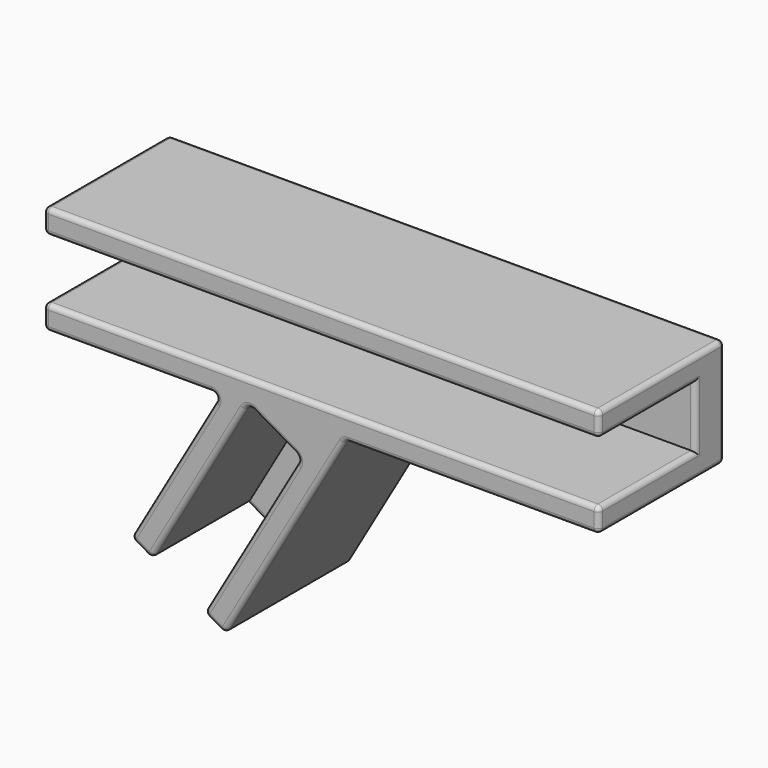
from build123d import *

# Parameters (mm, degrees)
F1_DEPTH      = 12.7
F0_W          = 58.42
F0_H          = 2.54
F0_H_2        = 6.35
F2_DEPTH      = 3.81
F4_T1_DEPTH   = 16.51
F4_T3_DEPTH   = 57.404
F4_T5_DEPTH   = 12.192
F4_T7_DEPTH   = 13.97
F4_T9_DEPTH   = 19.05
F4_T11_DEPTH  = 12.192
F4_T13_DEPTH  = 1.524
F4_T15_DEPTH  = 15.494
F4_T17_DEPTH  = 3.302
F4_T19_DEPTH  = 6.35
F4_T21_DEPTH  = 3.302
F4_T23_DEPTH  = 19.177
F4_T25_DEPTH  = 5.08
F4_T27_DEPTH  = 19.177
F4_T29_DEPTH  = 3.302
F4_T31_DEPTH  = 6.35
F4_S35_W      = 0.508
F4_S35_H      = 0.508
F4_T36_DEPTH  = 0.508
F4_S41_W      = 0.508
F4_S41_H      = 0.508
F4_T42_DEPTH  = 0.508
F4_S47_W      = 0.508
F4_S47_H      = 0.508
F4_T48_DEPTH  = 0.508
F4_S53_W      = 0.508
F4_S53_H      = 0.508
F4_T54_DEPTH  = 0.508
F4_S59_W      = 0.508
F4_S59_H      = 0.508
F4_T60_DEPTH  = 0.508
F4_S65_W      = 0.508
F4_S65_H      = 0.508
F4_T66_DEPTH  = 0.508
F4_S71_W      = 0.508
F4_S71_H      = 0.508
F4_T72_DEPTH  = 0.508
F4_S77_W      = 0.508
F4_S77_H      = 0.508
F4_T78_DEPTH  = 0.508
F4_S83_W      = 0.508
F4_S83_H      = 0.508
F4_T84_DEPTH  = 0.508
F4_S89_W      = 0.508
F4_S89_H      = 0.508
F4_T90_DEPTH  = 0.508
F4_T94_ANGLE  = 90
F4_T96_ANGLE  = 90
F4_T101_DEPTH = 13.462
F4_T105_DEPTH = 7.62
F4_T112_DEPTH = 13.462
F4_T116_DEPTH = 7.62
F4_T123_DEPTH = 13.462
F4_T127_DEPTH = 7.62
F4_T134_DEPTH = 7.62
F4_T138_DEPTH = 13.462
F4_T145_DEPTH = 13.462
F4_T149_DEPTH = 7.62
F4_T156_DEPTH = 7.62
F4_T160_DEPTH = 13.462
F4_T163_DEPTH = 17.1394104101
F4_T165_DEPTH = 17.4130046129
F4_T167_DEPTH = 24.5987060633
F4_T169_DEPTH = 25.8931866893
F4_T174_DEPTH = 0.508
F4_S179_W     = 0.508
F4_S179_H     = 0.508
F4_T180_DEPTH = 0.508
F4_S185_W     = 0.508
F4_S185_H     = 0.508
F4_T186_DEPTH = 0.508
F4_T192_DEPTH = 0.508
F4_S197_W     = 0.508
F4_S197_H     = 0.508
F4_T198_DEPTH = 0.508
F4_T204_DEPTH = 0.508
F4_T210_DEPTH = 0.508
F4_S215_W     = 0.508
F4_S215_H     = 0.508
F4_T216_DEPTH = 0.508
F4_T220_ANGLE = 120
F4_T222_ANGLE = 60
F4_T224_ANGLE = 60
F4_T226_ANGLE = 120


# Not quite as in the source:
# - a fillet or chamfer that OpenCascade refuses, or shapes differently, is made with other operations: its cross-section is extruded or revolved along the edge and cut away or added


with BuildPart() as f1:
    # F0 (on Front) → F1 (new body)
    with BuildSketch(Plane.XZ):
        with BuildLine():
            Line((29.21, -5.715), (29.21, -3.175))
            Line((29.21, -3.175), (-29.21, -3.175))
            Line((-29.21, -3.175), (-29.21, -5.715))
            Line((-29.21, -5.715), (-10.6827077797, -5.715))
            Line((-10.6827077797, -5.715), (-20.0831509913, -21.9970452561))
            Line((-20.0831509913, -21.9970452561), (-17.8834464656, -23.2670452561))
            Line((-17.8834464656, -23.2670452561), (-8.0409464656, -6.2193351826))
            ThreePointArc((-8.0409464656, -6.2193351826), (-7.6553704279, -5.9234722829), (-7.1735203342, -5.9869090512))
            Line((-7.1735203342, -5.9869090512), (-2.774111283, -8.5269090512))
            ThreePointArc((-2.774111283, -8.5269090512), (-2.4782483833, -8.912485089), (-2.5416851516, -9.3943351826))
            Line((-2.5416851516, -9.3943351826), (-12.3841851516, -26.4420452561))
            Line((-12.3841851516, -26.4420452561), (-10.184480626, -27.7120452561))
            Line((-10.184480626, -27.7120452561), (2.515519374, -5.715))
            Line((2.515519374, -5.715), (29.21, -5.715))
        make_face()
    extrude(amount=F1_DEPTH)



with BuildPart() as f1b:
    # F0 (on Front) → F1, piece 2 (new body)
    with BuildSketch(Plane.XZ):
        with Locations((0, 4.445)):
            Rectangle(F0_W, F0_H)
    extrude(amount=F1_DEPTH)


with BuildPart() as f1_1:
    add(f1.part)

    add(f1b.part)  # F2 merges F1b
    # F0 (on Front) → F2 (join)
    with BuildSketch(Plane.XZ):
        with Locations((0, 4.445)):
            Rectangle(F0_W, F0_H)
        Rectangle(F0_W, F0_H_2)
        with BuildLine():
            Line((-17.8834464656, -23.2670452561), (-12.3841851516, -26.4420452561))
            Line((-12.3841851516, -26.4420452561), (-2.5416851516, -9.3943351826))
            ThreePointArc((-2.5416851516, -9.3943351826), (-2.4782483833, -8.912485089), (-2.774111283, -8.5269090512))
            Line((-2.774111283, -8.5269090512), (-7.1735203342, -5.9869090512))
            ThreePointArc((-7.1735203342, -5.9869090512), (-7.6553704279, -5.9234722829), (-8.0409464656, -6.2193351826))
            Line((-8.0409464656, -6.2193351826), (-17.8834464656, -23.2670452561))
        make_face()
        with BuildLine():
            Line((29.21, -5.715), (29.21, -3.175))
            Line((29.21, -3.175), (-29.21, -3.175))
            Line((-29.21, -3.175), (-29.21, -5.715))
            Line((-29.21, -5.715), (-10.6827077797, -5.715))
            Line((-10.6827077797, -5.715), (-20.0831509913, -21.9970452561))
            Line((-20.0831509913, -21.9970452561), (-17.8834464656, -23.2670452561))
            Line((-17.8834464656, -23.2670452561), (-8.0409464656, -6.2193351826))
            ThreePointArc((-8.0409464656, -6.2193351826), (-7.6553704279, -5.9234722829), (-7.1735203342, -5.9869090512))
            Line((-7.1735203342, -5.9869090512), (-2.774111283, -8.5269090512))
            ThreePointArc((-2.774111283, -8.5269090512), (-2.4782483833, -8.912485089), (-2.5416851516, -9.3943351826))
            Line((-2.5416851516, -9.3943351826), (-12.3841851516, -26.4420452561))
            Line((-12.3841851516, -26.4420452561), (-10.184480626, -27.7120452561))
            Line((-10.184480626, -27.7120452561), (2.515519374, -5.715))
            Line((2.515519374, -5.715), (29.21, -5.715))
        make_face()
    extrude(amount=-F2_DEPTH)

    # F3: union 

    # F4: fillet of radius 0.508 on 43 edges, made by hand

    # F4_s2 → F4_t1 (join)
    with BuildSketch(Plane.XZ.offset(-3.81)):
        with BuildLine():
            ThreePointArc((2.8088133107, -5.715), (2.5548133107, -5.7830590949), (2.3688724056, -5.969))
            Line((2.3688724056, -5.969), (2.515519374, -5.715))
            Line((2.515519374, -5.715), (2.8088133107, -5.715))
        make_face()
        with BuildLine():
            ThreePointArc((-11.1226486848, -6.477), (-11.1226486848, -5.969), (-11.5625895899, -5.715))
            Line((-11.5625895899, -5.715), (-10.6827077797, -5.715))
            Line((-10.6827077797, -5.715), (-11.1226486848, -6.477))
        make_face()
    extrude(amount=F4_T1_DEPTH)

    # F4_s4 → F4_t3 (cut)
    with BuildSketch(Plane.YZ.offset(-28.702)):
        with BuildLine():
            ThreePointArc((3.302, 5.715), (3.6612102448, 5.5662102448), (3.81, 5.207))
            Line((3.81, 5.207), (3.81, 5.715))
            Line((3.81, 5.715), (3.302, 5.715))
        make_face()
        with BuildLine():
            ThreePointArc((-12.7, 5.207), (-12.5512102448, 5.5662102448), (-12.192, 5.715))
            Line((-12.192, 5.715), (-12.7, 5.715))
            Line((-12.7, 5.715), (-12.7, 5.207))
        make_face()
        with BuildLine():
            ThreePointArc((-12.192, 3.175), (-12.5512102448, 3.3237897552), (-12.7, 3.683))
            Line((-12.7, 3.683), (-12.7, 3.175))
            Line((-12.7, 3.175), (-12.192, 3.175))
        make_face()
        with BuildLine():
            ThreePointArc((-12.192, -3.175), (-12.5512102448, -3.3237897552), (-12.7, -3.683))
            Line((-12.7, -3.683), (-12.7, -3.175))
            Line((-12.7, -3.175), (-12.192, -3.175))
        make_face()
    extrude(amount=F4_T3_DEPTH, mode=Mode.SUBTRACT)

    # F4_s6 → F4_t5 (cut)
    with BuildSketch(Plane.XY.offset(-6.985)):
        with BuildLine():
            ThreePointArc((-29.21, 3.302), (-29.0612102448, 3.6612102448), (-28.702, 3.81))
            Line((-28.702, 3.81), (-29.21, 3.81))
            Line((-29.21, 3.81), (-29.21, 3.302))
        make_face()
        with BuildLine():
            ThreePointArc((29.21, 3.302), (29.0612102448, 3.6612102448), (28.702, 3.81))
            Line((28.702, 3.81), (29.21, 3.81))
            Line((29.21, 3.81), (29.21, 3.302))
        make_face()
    extrude(amount=F4_T5_DEPTH, mode=Mode.SUBTRACT)

    # F4_s8 → F4_t7 (cut)
    with BuildSketch(Plane(origin=(-6.6372155063, 0, 3.8319981592), x_dir=(0, 1, 0), z_dir=(0.8660254038, 0, -0.5))):
        with BuildLine():
            ThreePointArc((3.81, -28.5835754956), (3.6612102448, -28.9427857405), (3.302, -29.0915754956))
            Line((3.302, -29.0915754956), (3.81, -29.0915754956))
            Line((3.81, -29.0915754956), (3.81, -28.5835754956))
        make_face()
    extrude(amount=F4_T7_DEPTH, mode=Mode.SUBTRACT)

    # F4_s10 → F4_t9 (cut)
    with BuildSketch(Plane.XZ.offset(-5.08)):
        with BuildLine():
            ThreePointArc((-10.6244215311, -27.4580452561), (-10.2389414562, -27.5087946708), (-9.930480626, -27.272104351))
            Line((-9.930480626, -27.272104351), (-10.184480626, -27.7120452561))
            Line((-10.184480626, -27.7120452561), (-10.6244215311, -27.4580452561))
        make_face()
        with BuildLine():
            ThreePointArc((29.21, -5.207), (29.0612102448, -5.5662102448), (28.702, -5.715))
            Line((28.702, -5.715), (29.21, -5.715))
            Line((29.21, -5.715), (29.21, -5.207))
        make_face()
        with BuildLine():
            ThreePointArc((-29.21, -5.207), (-29.0612102448, -5.5662102448), (-28.702, -5.715))
            Line((-28.702, -5.715), (-29.21, -5.715))
            Line((-29.21, -5.715), (-29.21, -5.207))
        make_face()
        with BuildLine():
            ThreePointArc((-19.6432100861, -22.2510452561), (-19.8799004059, -21.9425844259), (-19.8291509913, -21.557104351))
            Line((-19.8291509913, -21.557104351), (-20.0831509913, -21.9970452561))
            Line((-20.0831509913, -21.9970452561), (-19.6432100861, -22.2510452561))
        make_face()
    extrude(amount=F4_T9_DEPTH, mode=Mode.SUBTRACT)

    # F4_s12 → F4_t11 (cut)
    with BuildSketch(Plane.XZ):
        with BuildLine():
            ThreePointArc((28.702, 3.175), (29.0612102448, 3.3237897552), (29.21, 3.683))
            Line((29.21, 3.683), (29.21, 3.175))
            Line((29.21, 3.175), (28.702, 3.175))
        make_face()
        with BuildLine():
            ThreePointArc((29.21, -3.683), (29.0612102448, -3.3237897552), (28.702, -3.175))
            Line((28.702, -3.175), (29.21, -3.175))
            Line((29.21, -3.175), (29.21, -3.683))
        make_face()
        with BuildLine():
            ThreePointArc((-28.702, 3.175), (-29.0612102448, 3.3237897552), (-29.21, 3.683))
            Line((-29.21, 3.683), (-29.21, 3.175))
            Line((-29.21, 3.175), (-28.702, 3.175))
        make_face()
        with BuildLine():
            ThreePointArc((-29.21, -3.683), (-29.0612102448, -3.3237897552), (-28.702, -3.175))
            Line((-28.702, -3.175), (-29.21, -3.175))
            Line((-29.21, -3.175), (-29.21, -3.683))
        make_face()
        with BuildLine():
            ThreePointArc((-18.3233873708, -23.0130452561), (-17.9379072959, -23.0637946708), (-17.6294464656, -22.827104351))
            Line((-17.6294464656, -22.827104351), (-17.8834464656, -23.2670452561))
            Line((-17.8834464656, -23.2670452561), (-18.3233873708, -23.0130452561))
        make_face()
        with BuildLine():
            ThreePointArc((-11.9442442465, -26.6960452561), (-12.1809345662, -26.3875844259), (-12.1301851516, -26.002104351))
            Line((-12.1301851516, -26.002104351), (-12.3841851516, -26.4420452561))
            Line((-12.3841851516, -26.4420452561), (-11.9442442465, -26.6960452561))
        make_face()
    extrude(amount=F4_T11_DEPTH, mode=Mode.SUBTRACT)

    # F4_s14 → F4_t13 (cut)
    with BuildSketch(Plane.XY.offset(3.683)):
        with BuildLine():
            ThreePointArc((29.21, -12.192), (29.0612102448, -12.5512102448), (28.702, -12.7))
            Line((28.702, -12.7), (29.21, -12.7))
            Line((29.21, -12.7), (29.21, -12.192))
        make_face()
        with BuildLine():
            ThreePointArc((-29.21, -12.192), (-29.0612102448, -12.5512102448), (-28.702, -12.7))
            Line((-28.702, -12.7), (-29.21, -12.7))
            Line((-29.21, -12.7), (-29.21, -12.192))
        make_face()
    extrude(amount=F4_T13_DEPTH, mode=Mode.SUBTRACT)

    # F4_s16 → F4_t15 (cut)
    with BuildSketch(Plane.XZ.offset(-3.302)):
        with BuildLine():
            ThreePointArc((29.21, 5.207), (29.0612102448, 5.5662102448), (28.702, 5.715))
            Line((28.702, 5.715), (29.21, 5.715))
            Line((29.21, 5.715), (29.21, 5.207))
        make_face()
        with BuildLine():
            ThreePointArc((-29.21, 5.207), (-29.0612102448, 5.5662102448), (-28.702, 5.715))
            Line((-28.702, 5.715), (-29.21, 5.715))
            Line((-29.21, 5.715), (-29.21, 5.207))
        make_face()
    extrude(amount=F4_T15_DEPTH, mode=Mode.SUBTRACT)

    # F4_s18 → F4_t17 (cut)
    with BuildSketch(Plane.XY.offset(-6.985)):
        with BuildLine():
            ThreePointArc((29.21, -12.192), (29.0612102448, -12.5512102448), (28.702, -12.7))
            Line((28.702, -12.7), (29.21, -12.7))
            Line((29.21, -12.7), (29.21, -12.192))
        make_face()
        with BuildLine():
            ThreePointArc((-29.21, -12.192), (-29.0612102448, -12.5512102448), (-28.702, -12.7))
            Line((-28.702, -12.7), (-29.21, -12.7))
            Line((-29.21, -12.7), (-29.21, -12.192))
        make_face()
    extrude(amount=F4_T17_DEPTH, mode=Mode.SUBTRACT)

    # F4_s20 → F4_t19 (cut)
    with BuildSketch(Plane.XY.offset(-3.175)):
        with BuildLine():
            ThreePointArc((29.21, 0.508), (29.0612102448, 0.1487897552), (28.702, 0))
            Line((28.702, 0), (29.21, 0))
            Line((29.21, 0), (29.21, 0.508))
        make_face()
        with BuildLine():
            ThreePointArc((-29.21, 0.508), (-29.0612102448, 0.1487897552), (-28.702, 0))
            Line((-28.702, 0), (-29.21, 0))
            Line((-29.21, 0), (-29.21, 0.508))
        make_face()
    extrude(amount=F4_T19_DEPTH, mode=Mode.SUBTRACT)

    # F4_s22 → F4_t21 (cut)
    with BuildSketch(Plane(origin=(-6.6372155063, 0, 3.8319981592), x_dir=(0, 1, 0), z_dir=(0.8660254038, 0, -0.5))):
        with BuildLine():
            ThreePointArc((-12.7, -28.5835754956), (-12.5512102448, -28.9427857405), (-12.192, -29.0915754956))
            Line((-12.192, -29.0915754956), (-12.7, -29.0915754956))
            Line((-12.7, -29.0915754956), (-12.7, -28.5835754956))
        make_face()
    extrude(amount=F4_T21_DEPTH, mode=Mode.SUBTRACT)

    # F4_s24 → F4_t23 (cut)
    with BuildSketch(Plane(origin=(-14.2917877478, 0, -24.7541025102), x_dir=(0, 1, 0), z_dir=(0.5, 0, 0.8660254038))):
        with BuildLine():
            ThreePointArc((-12.7, 4.3619963184), (-12.5512102448, 4.0027860736), (-12.192, 3.8539963184))
            Line((-12.192, 3.8539963184), (-12.7, 3.8539963184))
            Line((-12.7, 3.8539963184), (-12.7, 4.3619963184))
        make_face()
    extrude(amount=F4_T23_DEPTH, mode=Mode.SUBTRACT)

    # F4_s26 → F4_t25 (cut)
    with BuildSketch(Plane(origin=(-2.7877325864, 0, 1.6094981592), x_dir=(0, 1, 0), z_dir=(0.8660254038, 0, -0.5))):
        with BuildLine():
            ThreePointArc((-12.7, -8.2635754956), (-12.5512102448, -8.6227857405), (-12.192, -8.7715754956))
            Line((-12.192, -8.7715754956), (-12.7, -8.7715754956))
            Line((-12.7, -8.7715754956), (-12.7, -8.2635754956))
        make_face()
    extrude(amount=F4_T25_DEPTH, mode=Mode.SUBTRACT)

    # F4_s28 → F4_t27 (cut)
    with BuildSketch(Plane(origin=(-4.7032877478, 0, -8.1463333418), x_dir=(0, 1, 0), z_dir=(-0.5, 0, -0.8660254038))):
        with BuildLine():
            ThreePointArc((-12.7, 3.0040036816), (-12.5512102448, 2.6447934368), (-12.192, 2.4960036816))
            Line((-12.192, 2.4960036816), (-12.7, 2.4960036816))
            Line((-12.7, 2.4960036816), (-12.7, 3.0040036816))
        make_face()
    extrude(amount=F4_T27_DEPTH, mode=Mode.SUBTRACT)

    # F4_s30 → F4_t29 (cut)
    with BuildSketch(Plane(origin=(2.6015435013, 0, -1.5020018408), x_dir=(0, 1, 0), z_dir=(0.8660254038, 0, -0.5))):
        with BuildLine():
            ThreePointArc((-12.7, -28.5835754956), (-12.5512102448, -28.9427857405), (-12.192, -29.0915754956))
            Line((-12.192, -29.0915754956), (-12.7, -29.0915754956))
            Line((-12.7, -29.0915754956), (-12.7, -28.5835754956))
        make_face()
    extrude(amount=F4_T29_DEPTH, mode=Mode.SUBTRACT)

    # F4_s32 → F4_t31 (cut)
    with BuildSketch(Plane(origin=(-3.3376587178, 0, 1.9269981592), x_dir=(0, 1, 0), z_dir=(0.8660254038, 0, -0.5))):
        with BuildLine():
            ThreePointArc((0.508, -29.0915754956), (0.1487897552, -28.9427857405), (0, -28.5835754956))
            Line((0, -28.5835754956), (0, -29.0915754956))
            Line((0, -29.0915754956), (0.508, -29.0915754956))
        make_face()
    extrude(amount=F4_T31_DEPTH, mode=Mode.SUBTRACT)


with BuildPart() as f4_tool34:
    # F4_s35 → F4_t36 (new body)
    with BuildSketch(Plane.XZ.offset(-3.302)):
        with Locations((28.956, 5.461)):
            Rectangle(F4_S35_W, F4_S35_H)
    extrude(amount=-F4_T36_DEPTH)

    # F4_s37 → F4_t38 (revolve, cut)
    with BuildSketch(Plane(origin=(28.702, 3.302, 5.207), x_dir=(-0.7071067812, 0, -0.7071067812), z_dir=(0.7071067812, 0, -0.7071067812))):
        with BuildLine():
            ThreePointArc((0, -0.508), (0.508, 0), (0, 0.508))
            Line((0, 0.508), (0, -0.508))
        make_face()
    revolve(axis=Axis((28.702, 3.302, 5.207), (0, 1, 0)), mode=Mode.SUBTRACT)


with BuildPart() as f1_2:
    add(f1_1.part)

    # F4_t33: cut F4_tool34
    add(f4_tool34.part, mode=Mode.SUBTRACT)


with BuildPart() as f4_tool40:
    # F4_s41 → F4_t42 (new body)
    with BuildSketch(Plane.XZ.offset(-3.302)):
        with Locations((-28.956, 5.461)):
            Rectangle(F4_S41_W, F4_S41_H)
    extrude(amount=-F4_T42_DEPTH)

    # F4_s43 → F4_t44 (revolve, cut)
    with BuildSketch(Plane(origin=(-28.702, 3.302, 5.207), x_dir=(0.7071067812, 0, -0.7071067812), z_dir=(0.7071067812, 0, 0.7071067812))):
        with BuildLine():
            ThreePointArc((0, -0.508), (0.508, 0), (0, 0.508))
            Line((0, 0.508), (0, -0.508))
        make_face()
    revolve(axis=Axis((-28.702, 3.302, 5.207), (0, 1, 0)), mode=Mode.SUBTRACT)


with BuildPart() as f1_3:
    add(f1_2.part)

    # F4_t39: cut F4_tool40
    add(f4_tool40.part, mode=Mode.SUBTRACT)


with BuildPart() as f4_tool46:
    # F4_s47 → F4_t48 (new body)
    with BuildSketch(Plane.XY.offset(3.683)):
        with Locations((28.956, -12.446)):
            Rectangle(F4_S47_W, F4_S47_H)
    extrude(amount=-F4_T48_DEPTH)

    # F4_s49 → F4_t50 (revolve, cut)
    with BuildSketch(Plane(origin=(28.702, -12.192, 3.683), x_dir=(-0.7071067812, 0.7071067812, 0), z_dir=(-0.7071067812, -0.7071067812, 0))):
        with BuildLine():
            ThreePointArc((0, -0.508), (0.508, 0), (0, 0.508))
            Line((0, 0.508), (0, -0.508))
        make_face()
    revolve(axis=Axis((28.702, -12.192, 3.683), (0, 0, -1)), mode=Mode.SUBTRACT)


with BuildPart() as f1_4:
    add(f1_3.part)

    # F4_t45: cut F4_tool46
    add(f4_tool46.part, mode=Mode.SUBTRACT)


with BuildPart() as f4_tool52:
    # F4_s53 → F4_t54 (new body)
    with BuildSketch(Plane.YZ.offset(28.702)):
        with Locations((-12.446, 5.461)):
            Rectangle(F4_S53_W, F4_S53_H)
    extrude(amount=F4_T54_DEPTH)

    # F4_s55 → F4_t56 (revolve, cut)
    with BuildSketch(Plane(origin=(28.702, -12.192, 5.207), x_dir=(0, 0.7071067812, -0.7071067812), z_dir=(0, -0.7071067812, -0.7071067812))):
        with BuildLine():
            ThreePointArc((0, -0.508), (0.508, 0), (0, 0.508))
            Line((0, 0.508), (0, -0.508))
        make_face()
    revolve(axis=Axis((28.702, -12.192, 5.207), (1, 0, 0)), mode=Mode.SUBTRACT)


with BuildPart() as f1_5:
    add(f1_4.part)

    # F4_t51: cut F4_tool52
    add(f4_tool52.part, mode=Mode.SUBTRACT)


with BuildPart() as f4_tool58:
    # F4_s59 → F4_t60 (new body)
    with BuildSketch(Plane.YZ.offset(28.702)):
        with Locations((-12.446, -3.429)):
            Rectangle(F4_S59_W, F4_S59_H)
    extrude(amount=F4_T60_DEPTH)

    # F4_s61 → F4_t62 (revolve, cut)
    with BuildSketch(Plane(origin=(28.702, -12.192, -3.683), x_dir=(0, 0.7071067812, -0.7071067812), z_dir=(0, -0.7071067812, -0.7071067812))):
        with BuildLine():
            ThreePointArc((0, -0.508), (0.508, 0), (0, 0.508))
            Line((0, 0.508), (0, -0.508))
        make_face()
    revolve(axis=Axis((28.702, -12.192, -3.683), (1, 0, 0)), mode=Mode.SUBTRACT)


with BuildPart() as f1_6:
    add(f1_5.part)

    # F4_t57: cut F4_tool58
    add(f4_tool58.part, mode=Mode.SUBTRACT)


with BuildPart() as f4_tool64:
    # F4_s65 → F4_t66 (new body)
    with BuildSketch(Plane.YZ.offset(-28.702)):
        with Locations((-12.446, 5.461)):
            Rectangle(F4_S65_W, F4_S65_H)
    extrude(amount=-F4_T66_DEPTH)

    # F4_s67 → F4_t68 (revolve, cut)
    with BuildSketch(Plane(origin=(-28.702, -12.192, 5.207), x_dir=(0, 0.7071067812, -0.7071067812), z_dir=(0, 0.7071067812, 0.7071067812))):
        with BuildLine():
            ThreePointArc((0, -0.508), (0.508, 0), (0, 0.508))
            Line((0, 0.508), (0, -0.508))
        make_face()
    revolve(axis=Axis((-28.702, -12.192, 5.207), (-1, 0, 0)), mode=Mode.SUBTRACT)


with BuildPart() as f1_7:
    add(f1_6.part)

    # F4_t63: cut F4_tool64
    add(f4_tool64.part, mode=Mode.SUBTRACT)


with BuildPart() as f4_tool70:
    # F4_s71 → F4_t72 (new body)
    with BuildSketch(Plane.XY.offset(3.683)):
        with Locations((-28.956, -12.446)):
            Rectangle(F4_S71_W, F4_S71_H)
    extrude(amount=-F4_T72_DEPTH)

    # F4_s73 → F4_t74 (revolve, cut)
    with BuildSketch(Plane(origin=(-28.702, -12.192, 3.683), x_dir=(0.7071067812, 0.7071067812, 0), z_dir=(-0.7071067812, 0.7071067812, 0))):
        with BuildLine():
            ThreePointArc((0, -0.508), (0.508, 0), (0, 0.508))
            Line((0, 0.508), (0, -0.508))
        make_face()
    revolve(axis=Axis((-28.702, -12.192, 3.683), (0, 0, -1)), mode=Mode.SUBTRACT)


with BuildPart() as f1_8:
    add(f1_7.part)

    # F4_t69: cut F4_tool70
    add(f4_tool70.part, mode=Mode.SUBTRACT)


with BuildPart() as f4_tool76:
    # F4_s77 → F4_t78 (new body)
    with BuildSketch(Plane(origin=(-14.2917877478, 0, -24.7541025102), x_dir=(0, 1, 0), z_dir=(-0.5, 0, -0.8660254038))):
        with Locations((-12.446, -4.1079963184)):
            Rectangle(F4_S77_W, F4_S77_H)
    extrude(amount=F4_T78_DEPTH)

    # F4_s79 → F4_t80 (revolve, cut)
    with BuildSketch(Plane(origin=(-18.0693873708, -12.192, -22.573104351), x_dir=(-0.6123724357, 0.7071067812, 0.3535533906), z_dir=(-0.6123724357, -0.7071067812, 0.3535533906))):
        with BuildLine():
            ThreePointArc((0, -0.508), (0.508, 0), (0, 0.508))
            Line((0, 0.508), (0, -0.508))
        make_face()
    revolve(axis=Axis((-18.0693873708, -12.192, -22.573104351), (-0.5, 0, -0.8660254038)), mode=Mode.SUBTRACT)


with BuildPart() as f1_9:
    add(f1_8.part)

    # F4_t75: cut F4_tool76
    add(f4_tool76.part, mode=Mode.SUBTRACT)


with BuildPart() as f4_tool82:
    # F4_s83 → F4_t84 (new body)
    with BuildSketch(Plane(origin=(2.6015435013, 0, -1.5020018408), x_dir=(0, 1, 0), z_dir=(-0.8660254038, 0, 0.5))):
        with Locations((-12.446, 28.8375754956)):
            Rectangle(F4_S83_W, F4_S83_H)
    extrude(amount=F4_T84_DEPTH)

    # F4_s85 → F4_t86 (revolve, cut)
    with BuildSketch(Plane(origin=(-11.6902442465, -12.192, -26.256104351), x_dir=(0.3535533906, 0.7071067812, 0.6123724357), z_dir=(0.3535533906, -0.7071067812, 0.6123724357))):
        with BuildLine():
            ThreePointArc((0, -0.508), (0.508, 0), (0, 0.508))
            Line((0, 0.508), (0, -0.508))
        make_face()
    revolve(axis=Axis((-11.6902442465, -12.192, -26.256104351), (-0.8660254038, 0, 0.5)), mode=Mode.SUBTRACT)


with BuildPart() as f1_10:
    add(f1_9.part)

    # F4_t81: cut F4_tool82
    add(f4_tool82.part, mode=Mode.SUBTRACT)


with BuildPart() as f4_tool88:
    # F4_s89 → F4_t90 (new body)
    with BuildSketch(Plane.YZ.offset(-28.702)):
        with Locations((-12.446, -3.429)):
            Rectangle(F4_S89_W, F4_S89_H)
    extrude(amount=-F4_T90_DEPTH)

    # F4_s91 → F4_t92 (revolve, cut)
    with BuildSketch(Plane(origin=(-28.702, -12.192, -3.683), x_dir=(0, 0.7071067812, -0.7071067812), z_dir=(0, 0.7071067812, 0.7071067812))):
        with BuildLine():
            ThreePointArc((0, -0.508), (0.508, 0), (0, 0.508))
            Line((0, 0.508), (0, -0.508))
        make_face()
    revolve(axis=Axis((-28.702, -12.192, -3.683), (-1, 0, 0)), mode=Mode.SUBTRACT)


with BuildPart() as f1_11:
    add(f1_10.part)

    # F4_t87: cut F4_tool88
    add(f4_tool88.part, mode=Mode.SUBTRACT)

    # F4_s93 → F4_t94 (revolve, cut)
    with BuildSketch(Plane(origin=(-4.7032877478, 0, -8.1463333418), x_dir=(0, 1, 0), z_dir=(-0.5, 0, -0.8660254038))):
        with BuildLine():
            ThreePointArc((-12.7, -4.3619963184), (-12.5512102448, -4.0027860736), (-12.192, -3.8539963184))
            Line((-12.192, -3.8539963184), (-12.7, -3.8539963184))
            Line((-12.7, -3.8539963184), (-12.7, -4.3619963184))
        make_face()
    revolve(axis=Axis((-7.4910203342, -12.7, -6.5368351826), (0, 1, 0)), revolution_arc=F4_T94_ANGLE, mode=Mode.SUBTRACT)

    # F4_s95 → F4_t96 (revolve, cut)
    with BuildSketch(Plane(origin=(1.6116764648, 0, -0.9305018408), x_dir=(0, 1, 0), z_dir=(-0.8660254038, 0, 0.5))):
        with BuildLine():
            ThreePointArc((-12.7, 8.2635754956), (-12.5512102448, 8.6227857405), (-12.192, 8.7715754956))
            Line((-12.192, 8.7715754956), (-12.7, 8.7715754956))
            Line((-12.7, 8.7715754956), (-12.7, 8.2635754956))
        make_face()
    revolve(axis=Axis((-3.091611283, -12.7, -9.0768351826), (0, 1, 0)), revolution_arc=F4_T96_ANGLE, mode=Mode.SUBTRACT)


with BuildPart() as f4_tool99:
    # F4_s100 → F4_t101 (new body)
    with BuildSketch(Plane.XZ.offset(-1.27)):
        with BuildLine():
            ThreePointArc((28.702, 3.175), (29.0612102448, 3.3237897552), (29.21, 3.683))
            Line((29.21, 3.683), (29.21, 3.175))
            Line((29.21, 3.175), (28.702, 3.175))
        make_face()
    extrude(amount=F4_T101_DEPTH)

    split(bisect_by=Plane.XZ, keep=Keep.BOTTOM)


with BuildPart() as f4_tool103:
    # F4_s104 → F4_t105 (new body)
    with BuildSketch(Plane.XY.offset(-3.175)):
        with BuildLine():
            ThreePointArc((29.21, 0.508), (29.0612102448, 0.1487897552), (28.702, 0))
            Line((28.702, 0), (29.21, 0))
            Line((29.21, 0), (29.21, 0.508))
        make_face()
    extrude(amount=F4_T105_DEPTH)

    split(bisect_by=Plane.XY.offset(3.175), keep=Keep.TOP)


with BuildPart() as f4_tool99_1:
    add(f4_tool99.part)

    # F4_t107: intersect F4_tool103
    add(f4_tool103.part, mode=Mode.INTERSECT)


with BuildPart() as f1_12:
    add(f1_11.part)

    # F4_t97: cut F4_tool99
    add(f4_tool99_1.part, mode=Mode.SUBTRACT)


with BuildPart() as f4_tool110:
    # F4_s111 → F4_t112 (new body)
    with BuildSketch(Plane.XZ.offset(-1.27)):
        with BuildLine():
            ThreePointArc((29.21, -3.683), (29.0612102448, -3.3237897552), (28.702, -3.175))
            Line((28.702, -3.175), (29.21, -3.175))
            Line((29.21, -3.175), (29.21, -3.683))
        make_face()
    extrude(amount=F4_T112_DEPTH)

    split(bisect_by=Plane.XZ, keep=Keep.BOTTOM)


with BuildPart() as f4_tool114:
    # F4_s115 → F4_t116 (new body)
    with BuildSketch(Plane.XY.offset(-4.445)):
        with BuildLine():
            ThreePointArc((29.21, 0.508), (29.0612102448, 0.1487897552), (28.702, 0))
            Line((28.702, 0), (29.21, 0))
            Line((29.21, 0), (29.21, 0.508))
        make_face()
    extrude(amount=F4_T116_DEPTH)

    split(bisect_by=Plane.XY.offset(-3.175), keep=Keep.BOTTOM)


with BuildPart() as f4_tool110_1:
    add(f4_tool110.part)

    # F4_t118: intersect F4_tool114
    add(f4_tool114.part, mode=Mode.INTERSECT)


with BuildPart() as f1_13:
    add(f1_12.part)

    # F4_t108: cut F4_tool110
    add(f4_tool110_1.part, mode=Mode.SUBTRACT)


with BuildPart() as f4_tool121:
    # F4_s122 → F4_t123 (new body)
    with BuildSketch(Plane.XZ.offset(-1.27)):
        with BuildLine():
            ThreePointArc((-28.702, 3.175), (-29.0612102448, 3.3237897552), (-29.21, 3.683))
            Line((-29.21, 3.683), (-29.21, 3.175))
            Line((-29.21, 3.175), (-28.702, 3.175))
        make_face()
    extrude(amount=F4_T123_DEPTH)

    split(bisect_by=Plane.XZ, keep=Keep.BOTTOM)


with BuildPart() as f4_tool125:
    # F4_s126 → F4_t127 (new body)
    with BuildSketch(Plane.XY.offset(4.445)):
        with BuildLine():
            ThreePointArc((-29.21, 0.508), (-29.0612102448, 0.1487897552), (-28.702, 0))
            Line((-28.702, 0), (-29.21, 0))
            Line((-29.21, 0), (-29.21, 0.508))
        make_face()
    extrude(amount=-F4_T127_DEPTH)

    split(bisect_by=Plane.XY.offset(3.175), keep=Keep.TOP)


with BuildPart() as f4_tool121_1:
    add(f4_tool121.part)

    # F4_t129: intersect F4_tool125
    add(f4_tool125.part, mode=Mode.INTERSECT)


with BuildPart() as f1_14:
    add(f1_13.part)

    # F4_t119: cut F4_tool121
    add(f4_tool121_1.part, mode=Mode.SUBTRACT)


with BuildPart() as f4_tool132:
    # F4_s133 → F4_t134 (new body)
    with BuildSketch(Plane.XY.offset(3.175)):
        with BuildLine():
            ThreePointArc((-29.21, 0.508), (-29.0612102448, 0.1487897552), (-28.702, 0))
            Line((-28.702, 0), (-29.21, 0))
            Line((-29.21, 0), (-29.21, 0.508))
        make_face()
    extrude(amount=-F4_T134_DEPTH)

    split(bisect_by=Plane.XY.offset(-3.175), keep=Keep.BOTTOM)


with BuildPart() as f4_tool136:
    # F4_s137 → F4_t138 (new body)
    with BuildSketch(Plane.XZ.offset(-1.27)):
        with BuildLine():
            ThreePointArc((-29.21, -3.683), (-29.0612102448, -3.3237897552), (-28.702, -3.175))
            Line((-28.702, -3.175), (-29.21, -3.175))
            Line((-29.21, -3.175), (-29.21, -3.683))
        make_face()
    extrude(amount=F4_T138_DEPTH)

    split(bisect_by=Plane.XZ, keep=Keep.BOTTOM)


with BuildPart() as f4_tool132_1:
    add(f4_tool132.part)

    # F4_t140: intersect F4_tool136
    add(f4_tool136.part, mode=Mode.INTERSECT)


with BuildPart() as f1_15:
    add(f1_14.part)

    # F4_t130: cut F4_tool132
    add(f4_tool132_1.part, mode=Mode.SUBTRACT)


with BuildPart() as f4_tool143:
    # F4_s144 → F4_t145 (new body)
    with BuildSketch(Plane.XZ.offset(-1.27)):
        with BuildLine():
            ThreePointArc((-18.3233873708, -23.0130452561), (-17.9379072959, -23.0637946708), (-17.6294464656, -22.827104351))
            Line((-17.6294464656, -22.827104351), (-17.8834464656, -23.2670452561))
            Line((-17.8834464656, -23.2670452561), (-18.3233873708, -23.0130452561))
        make_face()
    extrude(amount=F4_T145_DEPTH)

    split(bisect_by=Plane.XZ, keep=Keep.BOTTOM)


with BuildPart() as f4_tool147:
    # F4_s148 → F4_t149 (new body)
    with BuildSketch(Plane(origin=(-4.4375109806, 0, 2.5619981592), x_dir=(0, 1, 0), z_dir=(0.8660254038, 0, -0.5))):
        with BuildLine():
            ThreePointArc((0.508, -29.0915754956), (0.1487897552, -28.9427857405), (0, -28.5835754956))
            Line((0, -28.5835754956), (0, -29.0915754956))
            Line((0, -29.0915754956), (0.508, -29.0915754956))
        make_face()
    extrude(amount=F4_T149_DEPTH)

    split(bisect_by=Plane(origin=(-3.3376587178, 0, 1.9269981592), x_dir=(0, 1, 0), z_dir=(-0.8660254038, 0, 0.5)), keep=Keep.TOP)


with BuildPart() as f4_tool143_1:
    add(f4_tool143.part)

    # F4_t151: intersect F4_tool147
    add(f4_tool147.part, mode=Mode.INTERSECT)


with BuildPart() as f1_16:
    add(f1_15.part)

    # F4_t141: cut F4_tool143
    add(f4_tool143_1.part, mode=Mode.SUBTRACT)


with BuildPart() as f4_tool154:
    # F4_s155 → F4_t156 (new body)
    with BuildSketch(Plane(origin=(-3.3376587178, 0, 1.9269981592), x_dir=(0, 1, 0), z_dir=(0.8660254038, 0, -0.5))):
        with BuildLine():
            ThreePointArc((0.508, -29.0915754956), (0.1487897552, -28.9427857405), (0, -28.5835754956))
            Line((0, -28.5835754956), (0, -29.0915754956))
            Line((0, -29.0915754956), (0.508, -29.0915754956))
        make_face()
    extrude(amount=F4_T156_DEPTH)

    split(bisect_by=Plane(origin=(2.1616025962, 0, -1.2480018408), x_dir=(0, 1, 0), z_dir=(0.8660254038, 0, -0.5)), keep=Keep.TOP)


with BuildPart() as f4_tool158:
    # F4_s159 → F4_t160 (new body)
    with BuildSketch(Plane.XZ.offset(-1.27)):
        with BuildLine():
            ThreePointArc((-11.9442442465, -26.6960452561), (-12.1809345662, -26.3875844259), (-12.1301851516, -26.002104351))
            Line((-12.1301851516, -26.002104351), (-12.3841851516, -26.4420452561))
            Line((-12.3841851516, -26.4420452561), (-11.9442442465, -26.6960452561))
        make_face()
    extrude(amount=F4_T160_DEPTH)

    split(bisect_by=Plane.XZ, keep=Keep.BOTTOM)


with BuildPart() as f4_tool154_1:
    add(f4_tool154.part)

    # F4_t162: intersect F4_tool158
    add(f4_tool158.part, mode=Mode.INTERSECT)


with BuildPart() as f1_17:
    add(f1_16.part)

    # F4_t152: cut F4_tool154
    add(f4_tool154_1.part, mode=Mode.SUBTRACT)

    # F4_s164 → F4_t163 (cut)
    with BuildSketch(Plane.YZ.offset(-28.702)):
        with BuildLine():
            ThreePointArc((3.81, -5.207), (3.6612102448, -5.5662102448), (3.302, -5.715))
            Line((3.302, -5.715), (3.81, -5.715))
            Line((3.81, -5.715), (3.81, -5.207))
        make_face()
        with BuildLine():
            ThreePointArc((-12.7, -5.207), (-12.5512102448, -5.5662102448), (-12.192, -5.715))
            Line((-12.192, -5.715), (-12.7, -5.715))
            Line((-12.7, -5.715), (-12.7, -5.207))
        make_face()
    extrude(amount=F4_T163_DEPTH, mode=Mode.SUBTRACT)

    # F4_s166 → F4_t165 (cut)
    with BuildSketch(Plane(origin=(-5.5852854414, 0, -9.6739981592), x_dir=(0, 1, 0), z_dir=(-0.5, 0, -0.8660254038))):
        with BuildLine():
            ThreePointArc((3.81, -5.8859963184), (3.6612102448, -6.2452065632), (3.302, -6.3939963184))
            Line((3.302, -6.3939963184), (3.81, -6.3939963184))
            Line((3.81, -6.3939963184), (3.81, -5.8859963184))
        make_face()
        with BuildLine():
            ThreePointArc((-12.7, -5.8859963184), (-12.5512102448, -6.2452065632), (-12.192, -6.3939963184))
            Line((-12.192, -6.3939963184), (-12.7, -6.3939963184))
            Line((-12.7, -6.3939963184), (-12.7, -5.8859963184))
        make_face()
    extrude(amount=F4_T165_DEPTH, mode=Mode.SUBTRACT)

    # F4_s168 → F4_t167 (cut)
    with BuildSketch(Plane(origin=(-14.2917877478, 0, -24.7541025102), x_dir=(0, 1, 0), z_dir=(0.5, 0, 0.8660254038))):
        with BuildLine():
            ThreePointArc((3.81, -4.5280036816), (3.6612102448, -4.8872139264), (3.302, -5.0360036816))
            Line((3.302, -5.0360036816), (3.81, -5.0360036816))
            Line((3.81, -5.0360036816), (3.81, -4.5280036816))
        make_face()
        with BuildLine():
            ThreePointArc((-12.7, -4.5280036816), (-12.5512102448, -4.8872139264), (-12.192, -5.0360036816))
            Line((-12.192, -5.0360036816), (-12.7, -5.0360036816))
            Line((-12.7, -5.0360036816), (-12.7, -4.5280036816))
        make_face()
    extrude(amount=F4_T167_DEPTH, mode=Mode.SUBTRACT)

    # F4_s170 → F4_t169 (cut)
    with BuildSketch(Plane.YZ.offset(2.8088133107)):
        with BuildLine():
            ThreePointArc((3.81, -5.207), (3.6612102448, -5.5662102448), (3.302, -5.715))
            Line((3.302, -5.715), (3.81, -5.715))
            Line((3.81, -5.715), (3.81, -5.207))
        make_face()
        with BuildLine():
            ThreePointArc((-12.7, -5.207), (-12.5512102448, -5.5662102448), (-12.192, -5.715))
            Line((-12.192, -5.715), (-12.7, -5.715))
            Line((-12.7, -5.715), (-12.7, -5.207))
        make_face()
    extrude(amount=F4_T169_DEPTH, mode=Mode.SUBTRACT)


with BuildPart() as f4_tool172:
    # F4_s173 → F4_t174 (new body)
    with BuildSketch(Plane.XZ.offset(12.192)):
        Polygon((-19.3892100861, -21.811104351), (-19.8291509913, -21.557104351), (-20.0831509913, -21.9970452561), (-19.6432100861, -22.2510452561), align=None)
    extrude(amount=F4_T174_DEPTH)

    # F4_s175 → F4_t176 (revolve, cut)
    with BuildSketch(Plane(origin=(-19.3892100861, -12.192, -21.811104351), x_dir=(0.9659258263, 0, 0.2588190451), z_dir=(0.2588190451, 0, -0.9659258263))):
        with BuildLine():
            ThreePointArc((0, -0.508), (0.508, 0), (0, 0.508))
            Line((0, 0.508), (0, -0.508))
        make_face()
    revolve(axis=Axis((-19.3892100861, -12.192, -21.811104351), (0, -1, 0)), mode=Mode.SUBTRACT)


with BuildPart() as f1_18:
    add(f1_17.part)

    # F4_t171: cut F4_tool172
    add(f4_tool172.part, mode=Mode.SUBTRACT)


with BuildPart() as f4_tool178:
    # F4_s179 → F4_t180 (new body)
    with BuildSketch(Plane.XZ.offset(12.192)):
        with Locations((-28.956, -5.461)):
            Rectangle(F4_S179_W, F4_S179_H)
    extrude(amount=F4_T180_DEPTH)

    # F4_s181 → F4_t182 (revolve, cut)
    with BuildSketch(Plane(origin=(-28.702, -12.192, -5.207), x_dir=(0.7071067812, 0, 0.7071067812), z_dir=(0.7071067812, 0, -0.7071067812))):
        with BuildLine():
            ThreePointArc((0, -0.508), (0.508, 0), (0, 0.508))
            Line((0, 0.508), (0, -0.508))
        make_face()
    revolve(axis=Axis((-28.702, -12.192, -5.207), (0, -1, 0)), mode=Mode.SUBTRACT)


with BuildPart() as f1_19:
    add(f1_18.part)

    # F4_t177: cut F4_tool178
    add(f4_tool178.part, mode=Mode.SUBTRACT)


with BuildPart() as f4_tool184:
    # F4_s185 → F4_t186 (new body)
    with BuildSketch(Plane.XZ.offset(12.192)):
        with Locations((28.956, -5.461)):
            Rectangle(F4_S185_W, F4_S185_H)
    extrude(amount=F4_T186_DEPTH)

    # F4_s187 → F4_t188 (revolve, cut)
    with BuildSketch(Plane(origin=(28.702, -12.192, -5.207), x_dir=(-0.7071067812, 0, 0.7071067812), z_dir=(0.7071067812, 0, 0.7071067812))):
        with BuildLine():
            ThreePointArc((0, -0.508), (0.508, 0), (0, 0.508))
            Line((0, 0.508), (0, -0.508))
        make_face()
    revolve(axis=Axis((28.702, -12.192, -5.207), (0, -1, 0)), mode=Mode.SUBTRACT)


with BuildPart() as f1_20:
    add(f1_19.part)

    # F4_t183: cut F4_tool184
    add(f4_tool184.part, mode=Mode.SUBTRACT)


with BuildPart() as f4_tool190:
    # F4_s191 → F4_t192 (new body)
    with BuildSketch(Plane.XZ.offset(12.192)):
        Polygon((-10.3704215311, -27.018104351), (-9.930480626, -27.272104351), (-10.184480626, -27.7120452561), (-10.6244215311, -27.4580452561), align=None)
    extrude(amount=F4_T192_DEPTH)

    # F4_s193 → F4_t194 (revolve, cut)
    with BuildSketch(Plane(origin=(-10.3704215311, -12.192, -27.018104351), x_dir=(-0.2588190451, 0, 0.9659258263), z_dir=(0.9659258263, 0, 0.2588190451))):
        with BuildLine():
            ThreePointArc((0, -0.508), (0.508, 0), (0, 0.508))
            Line((0, 0.508), (0, -0.508))
        make_face()
    revolve(axis=Axis((-10.3704215311, -12.192, -27.018104351), (0, -1, 0)), mode=Mode.SUBTRACT)


with BuildPart() as f1_21:
    add(f1_20.part)

    # F4_t189: cut F4_tool190
    add(f4_tool190.part, mode=Mode.SUBTRACT)


with BuildPart() as f4_tool196:
    # F4_s197 → F4_t198 (new body)
    with BuildSketch(Plane.XZ.offset(-3.302)):
        with Locations((28.956, -5.461)):
            Rectangle(F4_S197_W, F4_S197_H)
    extrude(amount=-F4_T198_DEPTH)

    # F4_s199 → F4_t200 (revolve, cut)
    with BuildSketch(Plane(origin=(28.702, 3.302, -5.207), x_dir=(-0.7071067812, 0, 0.7071067812), z_dir=(-0.7071067812, 0, -0.7071067812))):
        with BuildLine():
            ThreePointArc((0, -0.508), (0.508, 0), (0, 0.508))
            Line((0, 0.508), (0, -0.508))
        make_face()
    revolve(axis=Axis((28.702, 3.302, -5.207), (0, 1, 0)), mode=Mode.SUBTRACT)


with BuildPart() as f1_22:
    add(f1_21.part)

    # F4_t195: cut F4_tool196
    add(f4_tool196.part, mode=Mode.SUBTRACT)


with BuildPart() as f4_tool202:
    # F4_s203 → F4_t204 (new body)
    with BuildSketch(Plane.XZ.offset(-3.302)):
        Polygon((-10.3704215311, -27.018104351), (-9.930480626, -27.272104351), (-10.184480626, -27.7120452561), (-10.6244215311, -27.4580452561), align=None)
    extrude(amount=-F4_T204_DEPTH)

    # F4_s205 → F4_t206 (revolve, cut)
    with BuildSketch(Plane(origin=(-10.3704215311, 3.302, -27.018104351), x_dir=(-0.2588190451, 0, 0.9659258263), z_dir=(-0.9659258263, 0, -0.2588190451))):
        with BuildLine():
            ThreePointArc((0, -0.508), (0.508, 0), (0, 0.508))
            Line((0, 0.508), (0, -0.508))
        make_face()
    revolve(axis=Axis((-10.3704215311, 3.302, -27.018104351), (0, 1, 0)), mode=Mode.SUBTRACT)


with BuildPart() as f1_23:
    add(f1_22.part)

    # F4_t201: cut F4_tool202
    add(f4_tool202.part, mode=Mode.SUBTRACT)


with BuildPart() as f4_tool208:
    # F4_s209 → F4_t210 (new body)
    with BuildSketch(Plane.XZ.offset(-3.302)):
        Polygon((-19.3892100861, -21.811104351), (-19.8291509913, -21.557104351), (-20.0831509913, -21.9970452561), (-19.6432100861, -22.2510452561), align=None)
    extrude(amount=-F4_T210_DEPTH)

    # F4_s211 → F4_t212 (revolve, cut)
    with BuildSketch(Plane(origin=(-19.3892100861, 3.302, -21.811104351), x_dir=(0.9659258263, 0, 0.2588190451), z_dir=(-0.2588190451, 0, 0.9659258263))):
        with BuildLine():
            ThreePointArc((0, -0.508), (0.508, 0), (0, 0.508))
            Line((0, 0.508), (0, -0.508))
        make_face()
    revolve(axis=Axis((-19.3892100861, 3.302, -21.811104351), (0, 1, 0)), mode=Mode.SUBTRACT)


with BuildPart() as f1_24:
    add(f1_23.part)

    # F4_t207: cut F4_tool208
    add(f4_tool208.part, mode=Mode.SUBTRACT)


with BuildPart() as f4_tool214:
    # F4_s215 → F4_t216 (new body)
    with BuildSketch(Plane.XZ.offset(-3.302)):
        with Locations((-28.956, -5.461)):
            Rectangle(F4_S215_W, F4_S215_H)
    extrude(amount=-F4_T216_DEPTH)

    # F4_s217 → F4_t218 (revolve, cut)
    with BuildSketch(Plane(origin=(-28.702, 3.302, -5.207), x_dir=(0.7071067812, 0, 0.7071067812), z_dir=(-0.7071067812, 0, 0.7071067812))):
        with BuildLine():
            ThreePointArc((0, -0.508), (0.508, 0), (0, 0.508))
            Line((0, 0.508), (0, -0.508))
        make_face()
    revolve(axis=Axis((-28.702, 3.302, -5.207), (0, 1, 0)), mode=Mode.SUBTRACT)


with BuildPart() as f1_25:
    add(f1_24.part)

    # F4_t213: cut F4_tool214
    add(f4_tool214.part, mode=Mode.SUBTRACT)

    # F4_s219 → F4_t220 (revolve, cut)
    with BuildSketch(Plane(origin=(-5.5852854414, 0, -9.6739981592), x_dir=(0, 1, 0), z_dir=(-0.5, 0, -0.8660254038))):
        with BuildLine():
            ThreePointArc((-12.7, -5.8859963184), (-12.5512102448, -6.2452065632), (-12.192, -6.3939963184))
            Line((-12.192, -6.3939963184), (-12.7, -6.3939963184))
            Line((-12.7, -6.3939963184), (-12.7, -5.8859963184))
        make_face()
    revolve(axis=Axis((-11.5625895899, -12.7, -6.223), (0, -1, 0)), revolution_arc=F4_T220_ANGLE, mode=Mode.SUBTRACT)

    # F4_s221 → F4_t222 (revolve, cut)
    with BuildSketch(Plane.YZ.offset(2.8088133107)):
        with BuildLine():
            ThreePointArc((-12.7, -5.207), (-12.5512102448, -5.5662102448), (-12.192, -5.715))
            Line((-12.192, -5.715), (-12.7, -5.715))
            Line((-12.7, -5.715), (-12.7, -5.207))
        make_face()
    revolve(axis=Axis((2.8088133107, -12.7, -6.223), (0, -1, 0)), revolution_arc=F4_T222_ANGLE, mode=Mode.SUBTRACT)

    # F4_s223 → F4_t224 (revolve, cut)
    with BuildSketch(Plane.YZ.offset(2.8088133107)):
        with BuildLine():
            ThreePointArc((3.81, -5.207), (3.6612102448, -5.5662102448), (3.302, -5.715))
            Line((3.302, -5.715), (3.81, -5.715))
            Line((3.81, -5.715), (3.81, -5.207))
        make_face()
    revolve(axis=Axis((2.8088133107, 3.81, -6.223), (0, -1, 0)), revolution_arc=F4_T224_ANGLE, mode=Mode.SUBTRACT)

    # F4_s225 → F4_t226 (revolve, cut)
    with BuildSketch(Plane(origin=(-5.5852854414, 0, -9.6739981592), x_dir=(0, 1, 0), z_dir=(-0.5, 0, -0.8660254038))):
        with BuildLine():
            ThreePointArc((3.81, -5.8859963184), (3.6612102448, -6.2452065632), (3.302, -6.3939963184))
            Line((3.302, -6.3939963184), (3.81, -6.3939963184))
            Line((3.81, -6.3939963184), (3.81, -5.8859963184))
        make_face()
    revolve(axis=Axis((-11.5625895899, 3.81, -6.223), (0, -1, 0)), revolution_arc=F4_T226_ANGLE, mode=Mode.SUBTRACT)


solid = f1_25.part
